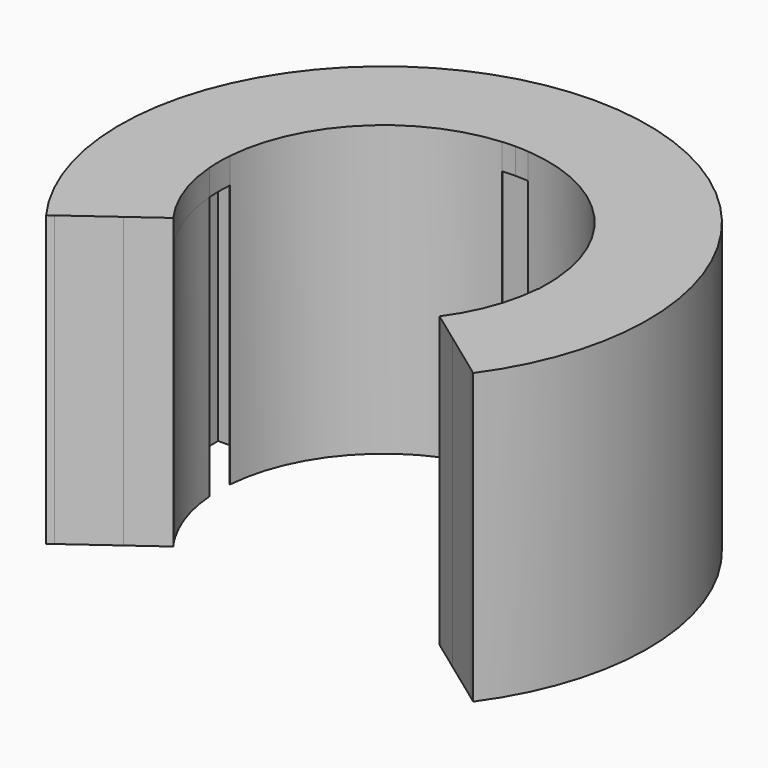
from build123d import *

# Parameters (mm, degrees)
F1_DEPTH = 10.16
F2_R     = 3
F4_DEPTH = 1
F6_DEPTH = 11.16
F8_DEPTH = 11.16


with BuildPart() as f1:
    # F0 (on Top) → F1 (new body)
    with BuildSketch(Plane.XY):
        with BuildLine():
            Line((2.4892, 8.382), (2.4892, 6.35))
            Line((2.4892, 6.35), (0.5, 6.35))
            ThreePointArc((0.5, 6.35), (0.4999030778, 6.340155572), (0.499612349, 6.3303149606))
            ThreePointArc((0.499612349, 6.3303149606), (4.4901280605, 4.4901280605), (6.3303149606, 0.499612349))
            ThreePointArc((6.3303149606, 0.499612349), (6.340155572, 0.4999030778), (6.35, 0.5))
            Line((6.35, 0.5), (6.35, 2.4892))
            Line((6.35, 2.4892), (8.382, 2.4892))
            Line((8.382, 2.4892), (8.382, -2.4892))
            Line((8.382, -2.4892), (6.35, -2.4892))
            Line((6.35, -2.4892), (6.35, -0.5))
            ThreePointArc((6.35, -0.5), (6.340155572, -0.4999030778), (6.3303149606, -0.499612349))
            ThreePointArc((6.3303149606, -0.499612349), (5.9570857831, -2.1990063604), (5.1366242038, -3.733308424))
            Line((5.1366242038, -3.733308424), (6.35, -4.6151923037))
            ThreePointArc((6.35, -4.6151923037), (6.5628814967, -4.3070972197), (6.760827121, -3.9892))
            Line((6.760827121, -3.9892), (9.882, -3.9892))
            Line((9.882, -3.9892), (9.882, 3.9892))
            Line((9.882, 3.9892), (6.760827121, 3.9892))
            ThreePointArc((6.760827121, 3.9892), (5.5507882323, 5.5507882323), (3.9892, 6.760827121))
            Line((3.9892, 6.760827121), (3.9892, 9.882))
            Line((3.9892, 9.882), (-3.9892, 9.882))
            Line((-3.9892, 9.882), (-3.9892, 6.760827121))
            ThreePointArc((-3.9892, 6.760827121), (-5.5507882323, 5.5507882323), (-6.760827121, 3.9892))
            Line((-6.760827121, 3.9892), (-9.882, 3.9892))
            Line((-9.882, 3.9892), (-9.882, -3.9892))
            Line((-9.882, -3.9892), (-6.760827121, -3.9892))
            ThreePointArc((-6.760827121, -3.9892), (-6.5628814967, -4.3070972197), (-6.35, -4.6151923037))
            Line((-6.35, -4.6151923037), (-5.1366242038, -3.733308424))
            ThreePointArc((-5.1366242038, -3.733308424), (-5.3088277076, -3.4840850121), (-5.4689493272, -3.2269324841))
            ThreePointArc((-5.4689493272, -3.2269324841), (-6.0551819306, -1.9123994841), (-6.3303149606, -0.499612349))
            ThreePointArc((-6.3303149606, -0.499612349), (-6.340155572, -0.4999030778), (-6.35, -0.5))
            Line((-6.35, -0.5), (-6.35, -2.4892))
            Line((-6.35, -2.4892), (-8.382, -2.4892))
            Line((-8.382, -2.4892), (-8.382, 2.4892))
            Line((-8.382, 2.4892), (-6.35, 2.4892))
            Line((-6.35, 2.4892), (-6.35, 0.5))
            ThreePointArc((-6.35, 0.5), (-6.340155572, 0.4999030778), (-6.3303149606, 0.499612349))
            ThreePointArc((-6.3303149606, 0.499612349), (-4.4901280605, 4.4901280605), (-0.499612349, 6.3303149606))
            ThreePointArc((-0.499612349, 6.3303149606), (-0.4999030778, 6.340155572), (-0.5, 6.35))
            Line((-0.5, 6.35), (-2.4892, 6.35))
            Line((-2.4892, 6.35), (-2.4892, 8.382))
            Line((-2.4892, 8.382), (2.4892, 8.382))
        make_face()
    extrude(amount=F1_DEPTH)

    # F2
    f2_edges = [f1.edges().sort_by_distance(p)[0] for p in [
        (-3.9892, 9.882, 5.08),
        (3.9892, 9.882, 5.08),
        (-9.882, 3.9892, 5.08),
        (-9.882, -3.9892, 5.08),
        (9.882, 3.9892, 5.08),
        (9.882, -3.9892, 5.08),
    ]]
    fillet(f2_edges, radius=F2_R)

    # F3 (on face) → F4 (join)
    with BuildSketch(Plane.XY.offset(10.16)):
        with BuildLine():
            ThreePointArc((-3.9892, 6.760827121), (-5.5507882323, 5.5507882323), (-6.760827121, 3.9892))
            Line((-6.760827121, 3.9892), (-6.882, 3.9892))
            ThreePointArc((-6.882, 3.9892), (-9.0033203436, 3.1105203436), (-9.882, 0.9892))
            Line((-9.882, 0.9892), (-9.882, -0.9892))
            ThreePointArc((-9.882, -0.9892), (-9.0033203436, -3.1105203436), (-6.882, -3.9892))
            Line((-6.882, -3.9892), (-6.760827121, -3.9892))
            ThreePointArc((-6.760827121, -3.9892), (-6.5628814967, -4.3070972197), (-6.35, -4.6151923037))
            Line((-6.35, -4.6151923037), (-5.1366242038, -3.733308424))
            ThreePointArc((-5.1366242038, -3.733308424), (-5.9570857831, -2.1990063604), (-6.3303149606, -0.499612349))
            ThreePointArc((-6.3303149606, -0.499612349), (-6.340155572, -0.4999030778), (-6.35, -0.5))
            Line((-6.35, -0.5), (-6.35, -2.4892))
            Line((-6.35, -2.4892), (-8.382, -2.4892))
            Line((-8.382, -2.4892), (-8.382, 2.4892))
            Line((-8.382, 2.4892), (-6.35, 2.4892))
            Line((-6.35, 2.4892), (-6.35, 0.5))
            ThreePointArc((-6.35, 0.5), (-6.340155572, 0.4999030778), (-6.3303149606, 0.499612349))
            ThreePointArc((-6.3303149606, 0.499612349), (-4.4901280605, 4.4901280605), (-0.499612349, 6.3303149606))
            ThreePointArc((-0.499612349, 6.3303149606), (-0.4999030778, 6.340155572), (-0.5, 6.35))
            Line((-0.5, 6.35), (-2.4892, 6.35))
            Line((-2.4892, 6.35), (-2.4892, 8.382))
            Line((-2.4892, 8.382), (2.4892, 8.382))
            Line((2.4892, 8.382), (2.4892, 6.35))
            Line((2.4892, 6.35), (0.5, 6.35))
            ThreePointArc((0.5, 6.35), (0.4999030778, 6.340155572), (0.499612349, 6.3303149606))
            ThreePointArc((0.499612349, 6.3303149606), (4.4901280605, 4.4901280605), (6.3303149606, 0.499612349))
            ThreePointArc((6.3303149606, 0.499612349), (6.340155572, 0.4999030778), (6.35, 0.5))
            Line((6.35, 0.5), (6.35, 2.4892))
            Line((6.35, 2.4892), (8.382, 2.4892))
            Line((8.382, 2.4892), (8.382, -2.4892))
            Line((8.382, -2.4892), (6.35, -2.4892))
            Line((6.35, -2.4892), (6.35, -0.5))
            ThreePointArc((6.35, -0.5), (6.340155572, -0.4999030778), (6.3303149606, -0.499612349))
            ThreePointArc((6.3303149606, -0.499612349), (5.9570857831, -2.1990063604), (5.1366242038, -3.733308424))
            Line((5.1366242038, -3.733308424), (6.35, -4.6151923037))
            ThreePointArc((6.35, -4.6151923037), (6.5628814967, -4.3070972197), (6.760827121, -3.9892))
            Line((6.760827121, -3.9892), (6.882, -3.9892))
            ThreePointArc((6.882, -3.9892), (9.0033203436, -3.1105203436), (9.882, -0.9892))
            Line((9.882, -0.9892), (9.882, 0.9892))
            ThreePointArc((9.882, 0.9892), (9.0033203436, 3.1105203436), (6.882, 3.9892))
            Line((6.882, 3.9892), (6.760827121, 3.9892))
            ThreePointArc((6.760827121, 3.9892), (5.5507882323, 5.5507882323), (3.9892, 6.760827121))
            Line((3.9892, 6.760827121), (3.9892, 6.882))
            ThreePointArc((3.9892, 6.882), (3.1105203436, 9.0033203436), (0.9892, 9.882))
            Line((0.9892, 9.882), (-0.9892, 9.882))
            ThreePointArc((-0.9892, 9.882), (-3.1105203436, 9.0033203436), (-3.9892, 6.882))
            Line((-3.9892, 6.882), (-3.9892, 6.760827121))
        make_face()
        with BuildLine():
            ThreePointArc((-6.35, -0.5), (-6.340155572, -0.4999030778), (-6.3303149606, -0.499612349))
            ThreePointArc((-6.3303149606, -0.499612349), (-6.35, 0), (-6.3303149606, 0.499612349))
            ThreePointArc((-6.3303149606, 0.499612349), (-6.340155572, 0.4999030778), (-6.35, 0.5))
            Line((-6.35, 0.5), (-6.35, 2.4892))
            Line((-6.35, 2.4892), (-8.382, 2.4892))
            Line((-8.382, 2.4892), (-8.382, -2.4892))
            Line((-8.382, -2.4892), (-6.35, -2.4892))
            Line((-6.35, -2.4892), (-6.35, -0.5))
        make_face()
        with BuildLine():
            ThreePointArc((-0.5, 6.35), (-0.4999030778, 6.340155572), (-0.499612349, 6.3303149606))
            ThreePointArc((-0.499612349, 6.3303149606), (-0.25, 6.3450768317), (0, 6.35))
            ThreePointArc((0, 6.35), (0.25, 6.3450768317), (0.499612349, 6.3303149606))
            ThreePointArc((0.499612349, 6.3303149606), (0.4999030778, 6.340155572), (0.5, 6.35))
            Line((0.5, 6.35), (2.4892, 6.35))
            Line((2.4892, 6.35), (2.4892, 8.382))
            Line((2.4892, 8.382), (-2.4892, 8.382))
            Line((-2.4892, 8.382), (-2.4892, 6.35))
            Line((-2.4892, 6.35), (-0.5, 6.35))
        make_face()
        with BuildLine():
            ThreePointArc((6.35, 0.5), (6.340155572, 0.4999030778), (6.3303149606, 0.499612349))
            ThreePointArc((6.3303149606, 0.499612349), (6.3450768317, 0.25), (6.35, 0))
            Line((6.35, 0), (6.35, -0.5))
            Line((6.35, -0.5), (6.35, -2.4892))
            Line((6.35, -2.4892), (8.382, -2.4892))
            Line((8.382, -2.4892), (8.382, 2.4892))
            Line((8.382, 2.4892), (6.35, 2.4892))
            Line((6.35, 2.4892), (6.35, 0.5))
        make_face()
    extrude(amount=F4_DEPTH)

    # F5 (on face) → F6 (join, through all)
    with BuildSketch(Plane(origin=(0, 0, 0), x_dir=(1, 0, 0), z_dir=(0, 0, -1))):
        with BuildLine():
            ThreePointArc((3.9892, -6.882), (3.3907514875, -8.6799294905), (1.8341663648, -9.7605468282))
            ThreePointArc((1.8341663648, -9.7605468282), (7.0225508414, -7.0225508414), (9.7605468282, -1.8341663648))
            ThreePointArc((9.7605468282, -1.8341663648), (8.6799294905, -3.3907514875), (6.882, -3.9892))
            Line((6.882, -3.9892), (6.760827121, -3.9892))
            ThreePointArc((6.760827121, -3.9892), (5.5507882323, -5.5507882323), (3.9892, -6.760827121))
            Line((3.9892, -6.760827121), (3.9892, -6.882))
        make_face()
        with BuildLine():
            ThreePointArc((6.882, 3.9892), (8.6799294905, 3.3907514875), (9.7605468282, 1.8341663648))
            ThreePointArc((9.7605468282, 1.8341663648), (9.1196479712, 3.9324879556), (8.0336694496, 5.8388865219))
            Line((8.0336694496, 5.8388865219), (6.35, 4.6151923037))
            ThreePointArc((6.35, 4.6151923037), (6.5628814967, 4.3070972197), (6.760827121, 3.9892))
            Line((6.760827121, 3.9892), (6.882, 3.9892))
        make_face()
        with BuildLine():
            ThreePointArc((-8.0336694496, 5.8388865219), (-9.1196479712, 3.9324879556), (-9.7605468282, 1.8341663648))
            ThreePointArc((-9.7605468282, 1.8341663648), (-8.6799294905, 3.3907514875), (-6.882, 3.9892))
            Line((-6.882, 3.9892), (-6.760827121, 3.9892))
            ThreePointArc((-6.760827121, 3.9892), (-6.5628814967, 4.3070972197), (-6.35, 4.6151923037))
            Line((-6.35, 4.6151923037), (-8.0336694496, 5.8388865219))
        make_face()
        with BuildLine():
            Line((-3.9892, -6.882), (-3.9892, -6.760827121))
            ThreePointArc((-3.9892, -6.760827121), (-5.5507882323, -5.5507882323), (-6.760827121, -3.9892))
            Line((-6.760827121, -3.9892), (-6.882, -3.9892))
            ThreePointArc((-6.882, -3.9892), (-8.6799294905, -3.3907514875), (-9.7605468282, -1.8341663648))
            ThreePointArc((-9.7605468282, -1.8341663648), (-7.0225508414, -7.0225508414), (-1.8341663648, -9.7605468282))
            ThreePointArc((-1.8341663648, -9.7605468282), (-3.3907514875, -8.6799294905), (-3.9892, -6.882))
        make_face()
    extrude(amount=-F6_DEPTH)

    # F7 (on face) → F8 (join, through all)
    with BuildSketch(Plane(origin=(0, 0, 0), x_dir=(1, 0, 0), z_dir=(0, 0, -1))):
        with BuildLine():
            Line((-7.8282044814, 5.6895541849), (-8.2391344177, 5.9882188588))
            ThreePointArc((-8.2391344177, 5.9882188588), (0, -10.1853866424), (8.2391344177, 5.9882188588))
            Line((8.2391344177, 5.9882188588), (7.8282044814, 5.6895541849))
            ThreePointArc((7.8282044814, 5.6895541849), (0, -9.6773866424), (-7.8282044814, 5.6895541849))
        make_face()
    extrude(amount=-F8_DEPTH)


solid = f1.part
